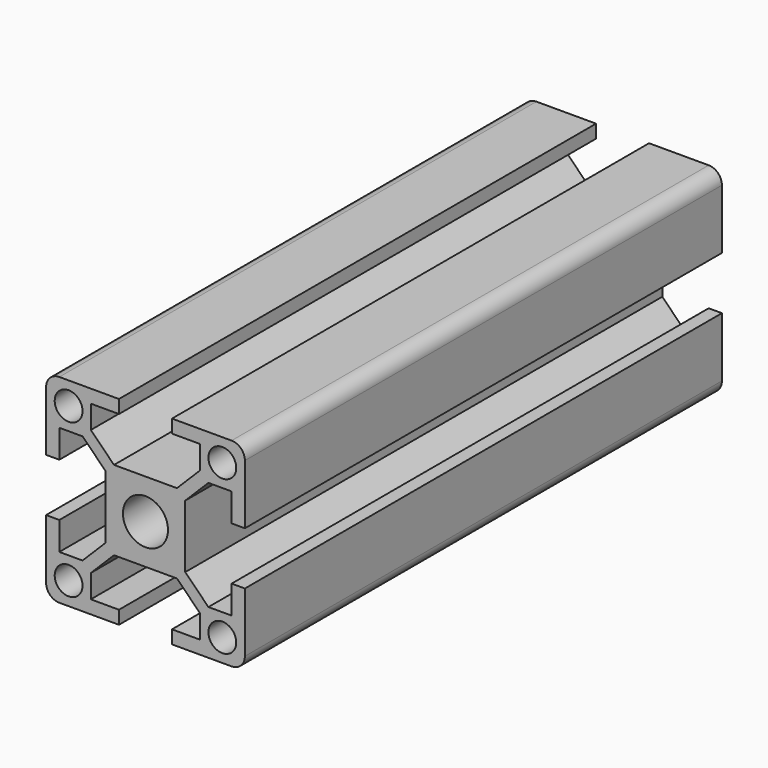
from build123d import *

# Parameters (mm, degrees)
F1_DEPTH = 90
F2_DEPTH = 400
F3_W     = 18.6485039899
F3_H     = 8
F3_W_2   = 19.9612321942
F3_R     = 3.4
F3_R_2   = 2.1
F4_DEPTH = 90
F5_R     = 2


# Not quite as in the source:
# - a pattern or mirror of a feature is missing from the dataset's text; its kind, count and spacing are read off the source's solid


with BuildPart() as f1:
    # F0 (on Front) → F1 (new body)
    with BuildSketch(Plane.XZ):
        Polygon((15, -15), (15, 15), (4, 15), (4, 13), (8.25, 13), (8.25, 9.5), (4.75, 6), (-4.75, 6), (-8.25, 9.5), (-8.25, 13), (-4, 13), (-4, 15), (-15, 15), (-15, -15), align=None)
        Polygon((4, 13), (4, 15), (-4, 15), (-4, 13), (-8.25, 13), (-8.25, 9.5), (-4.75, 6), (4.75, 6), (8.25, 9.5), (8.25, 13), align=None)
    extrude(amount=F1_DEPTH)

    # F0 (on Front) → F2 (cut)
    with BuildSketch(Plane.XZ):
        Polygon((4, 13), (4, 15), (-4, 15), (-4, 13), (-8.25, 13), (-8.25, 9.5), (-4.75, 6), (4.75, 6), (8.25, 9.5), (8.25, 13), align=None)
    f2 = extrude(amount=F2_DEPTH, mode=Mode.SUBTRACT)

    # F2_copies: F2 across plane
    add(f2.mirror(Plane(origin=(0, 0, 0), x_dir=(-1, 0, 0), z_dir=(0, 0, -1))), mode=Mode.SUBTRACT)

    # F3 (on face) → F4 (cut)
    with BuildSketch(Plane(origin=(0, 0, 0), x_dir=(-1, 0, 0), z_dir=(0, 1, 0))):
        Polygon((-6, 4.75), (-9.5, 8.25), (-13, 8.25), (-13, 4), (-13, -4), (-13, -8.25), (-9.5, -8.25), (-6, -4.75), align=None)
        with Locations((-22.3242519949, 0)):
            Rectangle(F3_W, F3_H)
        Polygon((13, 8.25), (9.5, 8.25), (6, 4.75), (6, -4.75), (9.5, -8.25), (13, -8.25), (13, -4), (13, 4), align=None)
        with Locations((22.9806160971, 0)):
            Rectangle(F3_W_2, F3_H)
        Circle(F3_R)
        with Locations((-11.6, 11.6)):
            Circle(F3_R_2)
        with Locations((-11.6, -11.6)):
            Circle(F3_R_2)
        with Locations((11.6, -11.6)):
            Circle(F3_R_2)
        with Locations((11.6, 11.6)):
            Circle(F3_R_2)
    extrude(amount=-F4_DEPTH, mode=Mode.SUBTRACT)

    # F5
    f5_edges = [f1.edges().sort_by_distance(p)[0] for p in [
        (-15, -45, 15),
        (-15, -45, -15),
        (15, -45, -15),
        (15, -45, 15),
    ]]
    fillet(f5_edges, radius=F5_R)


solid = f1.part
